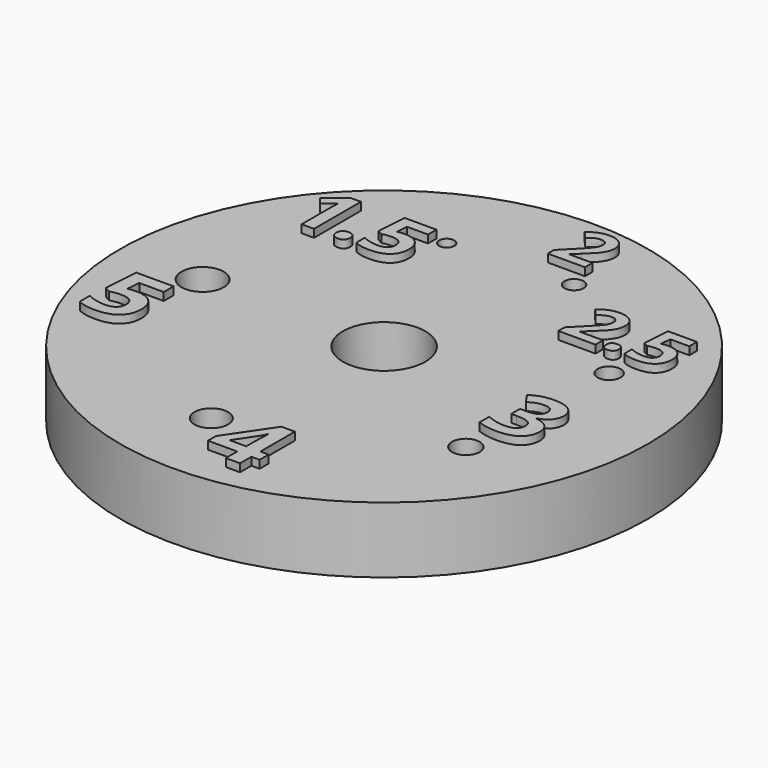
from build123d import *

# Parameters (mm, degrees)
F0_R           = 40
F0_R_2         = 2.55
F0_R_3         = 2.1
F0_R_4         = 3.2
F0_R_5         = 1.15
F0_R_6         = 1.75
F0_R_7         = 1.45
F1_DEPTH       = 10
F3_D           = 6.6
F3_CBORE_D     = 12.5
F3_CBORE_DEPTH = 7
F4_TEXT_SIZE   = 14.5525593931
F4_TEXT_SIZE_2 = 14.5525568061
F4_TEXT_SIZE_3 = 14.3171352748
F4_TEXT_SIZE_4 = 11.2665002234
F4_TEXT_SIZE_5 = 11.2665015169
F4_TEXT_SIZE_6 = 12.4400869633
F5_DEPTH       = 1.2


# Not quite as in the source:
# - Text() gives the source's letters only with a copy of the font that has no kerning and outlines rounded to 1/6400 em; it was checked with that copy


with BuildPart() as f1:
    # F0 (on Top) → F1 (new body)
    with BuildSketch(Plane.XY):
        Circle(F0_R)
        with Locations((-4.4807056229, -27.1325132843)):
            Circle(F0_R_2, mode=Mode.SUBTRACT)
        with Locations((23.6388818001, -14.0518065473)):
            Circle(F0_R_3, mode=Mode.SUBTRACT)
        with Locations((-27.5, 0)):
            Circle(F0_R_4, mode=Mode.SUBTRACT)
        with Locations((-10.753800456, 25.3101911441)):
            Circle(F0_R_5, mode=Mode.SUBTRACT)
        with Locations((25.0804742477, 11.279176012)):
            Circle(F0_R_6, mode=Mode.SUBTRACT)
        with Locations((7.6612837808, 26.4112614396)):
            Circle(F0_R_7, mode=Mode.SUBTRACT)
    extrude(amount=F1_DEPTH)

    # F3 (through all)
    with Locations(Plane.XY.offset(10)):
        with Locations((0, 0)):
            CounterBoreHole(F3_D / 2, F3_CBORE_D / 2, F3_CBORE_DEPTH)

    # F4 (on face) → F5 (join)
    with BuildSketch(Plane.XY.offset(10)):
        with Locations((-34.5838665962, -15.7162565738)):
            Text('5', F4_TEXT_SIZE, font='Open Sans', font_style=FontStyle.BOLD, text_align=(TextAlign.LEFT, TextAlign.BOTTOM))
        with Locations((0, -35.8269512653)):
            Text('4', F4_TEXT_SIZE_2, font='Open Sans', font_style=FontStyle.BOLD, text_align=(TextAlign.LEFT, TextAlign.BOTTOM))
        with Locations((21.8612812459, -10.3083373979)):
            Text('3', F4_TEXT_SIZE_3, font='Open Sans', font_style=FontStyle.BOLD, text_align=(TextAlign.LEFT, TextAlign.BOTTOM))
        with Locations((14.594390057, 14.1962924972)):
            Text('2.5', F4_TEXT_SIZE_4, font='Open Sans', font_style=FontStyle.BOLD, text_align=(TextAlign.LEFT, TextAlign.BOTTOM))
        with Locations((1.2435921235, 28.8990717381)):
            Text('2', F4_TEXT_SIZE_5, font='Open Sans', font_style=FontStyle.BOLD, text_align=(TextAlign.LEFT, TextAlign.BOTTOM))
        with Locations((-29.0069524199, 16.5622588247)):
            Text('1.5', F4_TEXT_SIZE_6, font='Open Sans', font_style=FontStyle.BOLD, text_align=(TextAlign.LEFT, TextAlign.BOTTOM))
    extrude(amount=F5_DEPTH)


solid = f1.part
